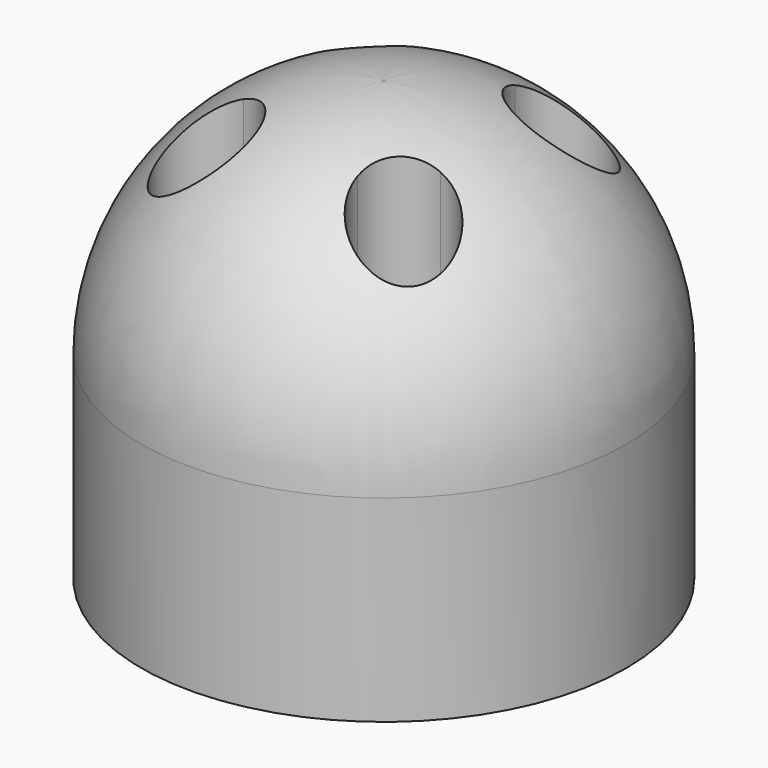
from build123d import *

# Parameters (mm, degrees)
F0_R     = 11.075
F1_DEPTH = 20
F3_DEPTH = 20.001
F5_DEPTH = 13.69


# Not quite as in the source:
# - a fillet or chamfer that OpenCascade refuses, or shapes differently, is made with other operations: its cross-section is extruded or revolved along the edge and cut away or added


with BuildPart() as f1:
    # F0 (on Top) → F1 (new body)
    with BuildSketch(Plane.XY):
        Circle(F0_R)
    extrude(amount=F1_DEPTH)

    # F2 (on face) → F3 (cut, through all)
    with BuildSketch(Plane.XY.offset(20)):
        with BuildLine():
            Line((4.5, 4.5), (3.5, 4.5))
            ThreePointArc((3.5, 4.5), (3.7928932188, 3.7928932188), (4.5, 3.5))
            Line((4.5, 3.5), (4.5, 4.5))
        make_face()
        with BuildLine():
            Line((-4.5, 4.5), (-3.5, 4.5))
            ThreePointArc((-3.5, 4.5), (-5.2071067812, 5.2071067812), (-4.5, 3.5))
            Line((-4.5, 3.5), (-4.5, 4.5))
        make_face()
        with BuildLine():
            ThreePointArc((-4.5, 3.5), (-3.7928932188, 3.7928932188), (-3.5, 4.5))
            Line((-3.5, 4.5), (-4.5, 4.5))
            Line((-4.5, 4.5), (-4.5, 3.5))
        make_face()
        with BuildLine():
            Line((4.5, -4.5), (4.5, -3.5))
            ThreePointArc((4.5, -3.5), (3.7928932188, -3.7928932188), (3.5, -4.5))
            Line((3.5, -4.5), (4.5, -4.5))
        make_face()
        with BuildLine():
            ThreePointArc((5.5, -4.5), (5.2071067812, -3.7928932188), (4.5, -3.5))
            Line((4.5, -3.5), (4.5, -4.5))
            Line((4.5, -4.5), (3.5, -4.5))
            ThreePointArc((3.5, -4.5), (4.5, -5.5), (5.5, -4.5))
        make_face()
        with BuildLine():
            ThreePointArc((-3.5, -4.5), (-3.7928932188, -3.7928932188), (-4.5, -3.5))
            Line((-4.5, -3.5), (-4.5, -4.5))
            Line((-4.5, -4.5), (-3.5, -4.5))
        make_face()
        with BuildLine():
            Line((-4.5, -4.5), (-4.5, -3.5))
            ThreePointArc((-4.5, -3.5), (-5.2071067812, -5.2071067812), (-3.5, -4.5))
            Line((-3.5, -4.5), (-4.5, -4.5))
        make_face()
        with BuildLine():
            ThreePointArc((5.5, 4.5), (4.5, 5.5), (3.5, 4.5))
            Line((3.5, 4.5), (4.5, 4.5))
            Line((4.5, 4.5), (4.5, 3.5))
            ThreePointArc((4.5, 3.5), (5.2071067812, 3.7928932188), (5.5, 4.5))
        make_face()
    extrude(amount=-F3_DEPTH, mode=Mode.SUBTRACT)

    # F4 (on face) → F5 (cut)
    with BuildSketch(Plane.XY.offset(20)):
        with BuildLine():
            ThreePointArc((-4.5, -3.5), (-3.7928932188, -3.7928932188), (-3.5, -4.5))
            Line((-3.5, -4.5), (-2.4, -4.5))
            ThreePointArc((-2.4, -4.5), (-3.0150757595, -3.0150757595), (-4.5, -2.4))
            Line((-4.5, -2.4), (-4.5, -3.5))
        make_face()
        with BuildLine():
            Line((-2.4, -4.5), (-3.5, -4.5))
            ThreePointArc((-3.5, -4.5), (-5.2071067812, -5.2071067812), (-4.5, -3.5))
            Line((-4.5, -3.5), (-4.5, -2.4))
            ThreePointArc((-4.5, -2.4), (-5.9849242405, -5.9849242405), (-2.4, -4.5))
        make_face()
        with BuildLine():
            ThreePointArc((4.5, -2.4), (3.0150757595, -3.0150757595), (2.4, -4.5))
            Line((2.4, -4.5), (3.5, -4.5))
            ThreePointArc((3.5, -4.5), (3.7928932188, -3.7928932188), (4.5, -3.5))
            Line((4.5, -3.5), (4.5, -2.4))
        make_face()
        with BuildLine():
            Line((3.5, -4.5), (2.4, -4.5))
            ThreePointArc((2.4, -4.5), (4.5, -6.6), (6.6, -4.5))
            ThreePointArc((6.6, -4.5), (5.9849242405, -3.0150757595), (4.5, -2.4))
            Line((4.5, -2.4), (4.5, -3.5))
            ThreePointArc((4.5, -3.5), (5.2071067812, -3.7928932188), (5.5, -4.5))
            ThreePointArc((5.5, -4.5), (4.5, -5.5), (3.5, -4.5))
        make_face()
        with BuildLine():
            ThreePointArc((-2.4, 4.5), (-5.9849242405, 5.9849242405), (-4.5, 2.4))
            Line((-4.5, 2.4), (-4.5, 3.5))
            ThreePointArc((-4.5, 3.5), (-5.2071067812, 5.2071067812), (-3.5, 4.5))
            Line((-3.5, 4.5), (-2.4, 4.5))
        make_face()
        with BuildLine():
            Line((-4.5, 3.5), (-4.5, 2.4))
            ThreePointArc((-4.5, 2.4), (-3.0150757595, 3.0150757595), (-2.4, 4.5))
            Line((-2.4, 4.5), (-3.5, 4.5))
            ThreePointArc((-3.5, 4.5), (-3.7928932188, 3.7928932188), (-4.5, 3.5))
        make_face()
        with BuildLine():
            ThreePointArc((2.4, 4.5), (3.0150757595, 3.0150757595), (4.5, 2.4))
            Line((4.5, 2.4), (4.5, 3.5))
            ThreePointArc((4.5, 3.5), (3.7928932188, 3.7928932188), (3.5, 4.5))
            Line((3.5, 4.5), (2.4, 4.5))
        make_face()
        with BuildLine():
            Line((4.5, 3.5), (4.5, 2.4))
            ThreePointArc((4.5, 2.4), (5.9849242405, 3.0150757595), (6.6, 4.5))
            ThreePointArc((6.6, 4.5), (4.5, 6.6), (2.4, 4.5))
            Line((2.4, 4.5), (3.5, 4.5))
            ThreePointArc((3.5, 4.5), (4.5, 5.5), (5.5, 4.5))
            ThreePointArc((5.5, 4.5), (5.2071067812, 3.7928932188), (4.5, 3.5))
        make_face()
        with BuildLine():
            Line((-4.5, -3.5), (-4.5, -4.5))
            Line((-4.5, -4.5), (-3.5, -4.5))
            ThreePointArc((-3.5, -4.5), (-3.7928932188, -3.7928932188), (-4.5, -3.5))
        make_face()
        with BuildLine():
            Line((-3.5, -4.5), (-4.5, -4.5))
            Line((-4.5, -4.5), (-4.5, -3.5))
            ThreePointArc((-4.5, -3.5), (-5.2071067812, -5.2071067812), (-3.5, -4.5))
        make_face()
        with BuildLine():
            ThreePointArc((4.5, -3.5), (3.7928932188, -3.7928932188), (3.5, -4.5))
            Line((3.5, -4.5), (4.5, -4.5))
            Line((4.5, -4.5), (4.5, -3.5))
        make_face()
        with BuildLine():
            Line((4.5, -4.5), (3.5, -4.5))
            ThreePointArc((3.5, -4.5), (4.5, -5.5), (5.5, -4.5))
            ThreePointArc((5.5, -4.5), (5.2071067812, -3.7928932188), (4.5, -3.5))
            Line((4.5, -3.5), (4.5, -4.5))
        make_face()
        with BuildLine():
            ThreePointArc((-3.5, 4.5), (-5.2071067812, 5.2071067812), (-4.5, 3.5))
            Line((-4.5, 3.5), (-4.5, 4.5))
            Line((-4.5, 4.5), (-3.5, 4.5))
        make_face()
        with BuildLine():
            Line((-4.5, 4.5), (-4.5, 3.5))
            ThreePointArc((-4.5, 3.5), (-3.7928932188, 3.7928932188), (-3.5, 4.5))
            Line((-3.5, 4.5), (-4.5, 4.5))
        make_face()
        with BuildLine():
            ThreePointArc((3.5, 4.5), (3.7928932188, 3.7928932188), (4.5, 3.5))
            Line((4.5, 3.5), (4.5, 4.5))
            Line((4.5, 4.5), (3.5, 4.5))
        make_face()
        with BuildLine():
            Line((4.5, 4.5), (4.5, 3.5))
            ThreePointArc((4.5, 3.5), (5.2071067812, 3.7928932188), (5.5, 4.5))
            ThreePointArc((5.5, 4.5), (4.5, 5.5), (3.5, 4.5))
            Line((3.5, 4.5), (4.5, 4.5))
        make_face()
    extrude(amount=-F5_DEPTH, mode=Mode.SUBTRACT)

    # F6: fillet of radius 11 on 1 edges, made by hand

    # F6_s1 → F6_t2 (revolve, cut)
    with BuildSketch(Plane.XZ):
        with BuildLine():
            ThreePointArc((11.075, 9), (7.8531745931, 16.7781745931), (0.075, 20))
            Line((0.075, 20), (11.075, 20))
            Line((11.075, 20), (11.075, 9))
        make_face()
    revolve(axis=Axis((0, 0, 20), (0, 0, 1)), mode=Mode.SUBTRACT)


solid = f1.part
